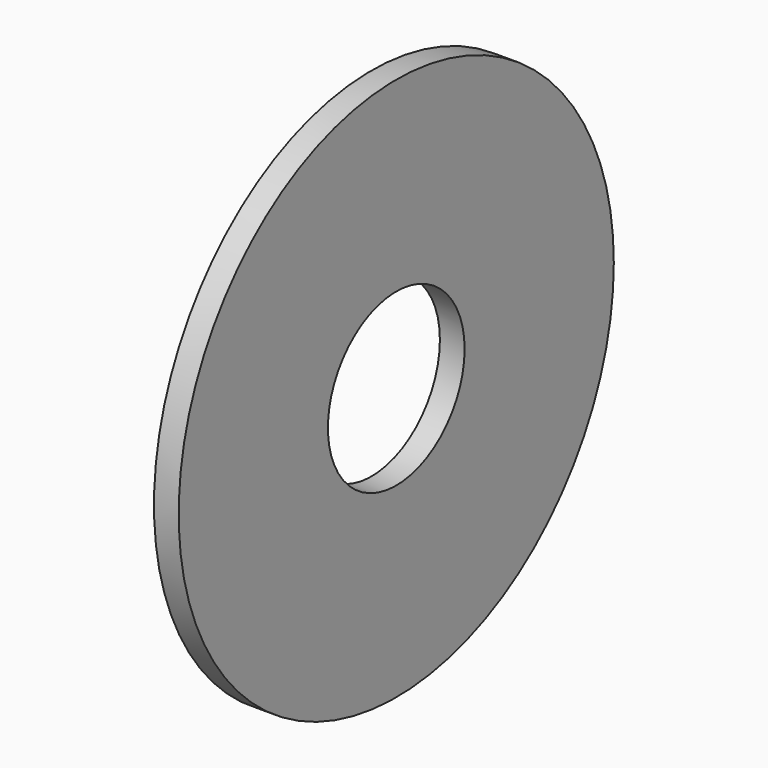
from build123d import *

# Parameters (mm, degrees)
F1_R     = 69.85
F1_R_2   = 21.9433592394
F2_DEPTH = 6.35


# Not quite as in the source:
# - a variable given as a bare number and used for a length is read in inches; the dataset says mm whatever the document's units were


with BuildPart() as f2:
    # F1 (on Right) → F2 (new body)
    with BuildSketch(Plane.YZ):
        Circle(F1_R)
        Circle(F1_R_2, mode=Mode.SUBTRACT)
    extrude(amount=F2_DEPTH)


solid = f2.part
